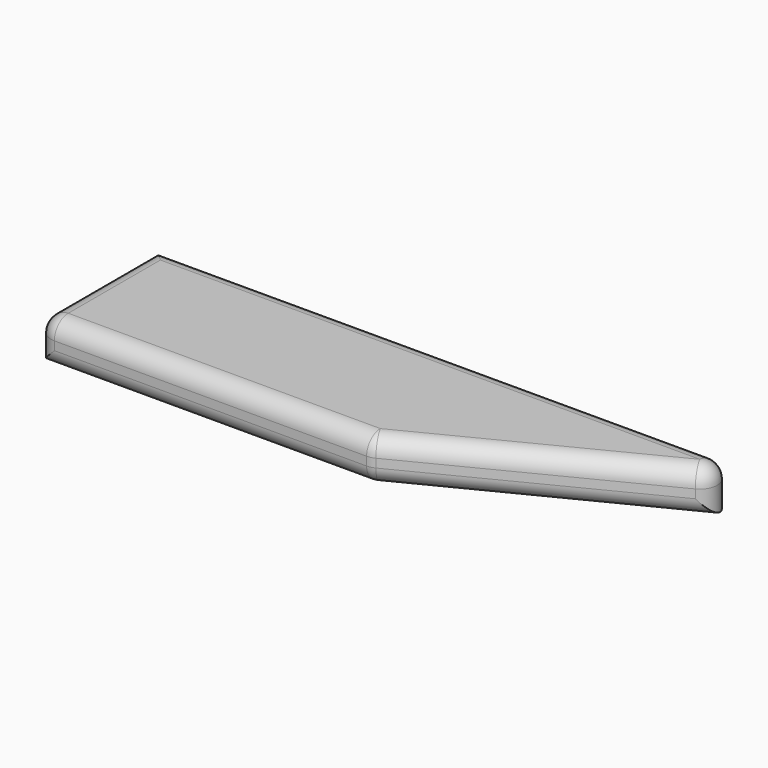
from build123d import *

# Parameters (mm, degrees)
F1_DEPTH = 12.7
F2_R     = 5.08


# Not quite as in the source:
# - the program builds the solid bodies; features that only make, move or delete a surface that nothing else refers to are left out


with BuildPart() as f1:
    # F0 (on Top) → F1 (new body)
    with BuildSketch(Plane.XY):
        Polygon((140.0786787271, 19.4519720972), (-44.8985807598, 19.4519720972), (-44.8985807598, -24.5902296156), (53.217664361, -24.5902296156), align=None)
    extrude(amount=F1_DEPTH)

    # F2
    f2_edges = [f1.edges().sort_by_distance(p)[0] for p in [
        (96.648172, -2.569129, 12.7),
        (47.590049, 19.451972, 12.7),
        (-44.898581, -2.569129, 12.7),
        (4.159542, -24.59023, 12.7),
        (-44.898581, -24.59023, 6.35),
        (53.217664, -24.59023, 6.35),
        (4.159542, -24.59023, 0),
        (140.078679, 19.451972, 6.35),
        (96.648172, -2.569129, 0),
    ]]
    fillet(f2_edges, radius=F2_R)


solid = f1.part
